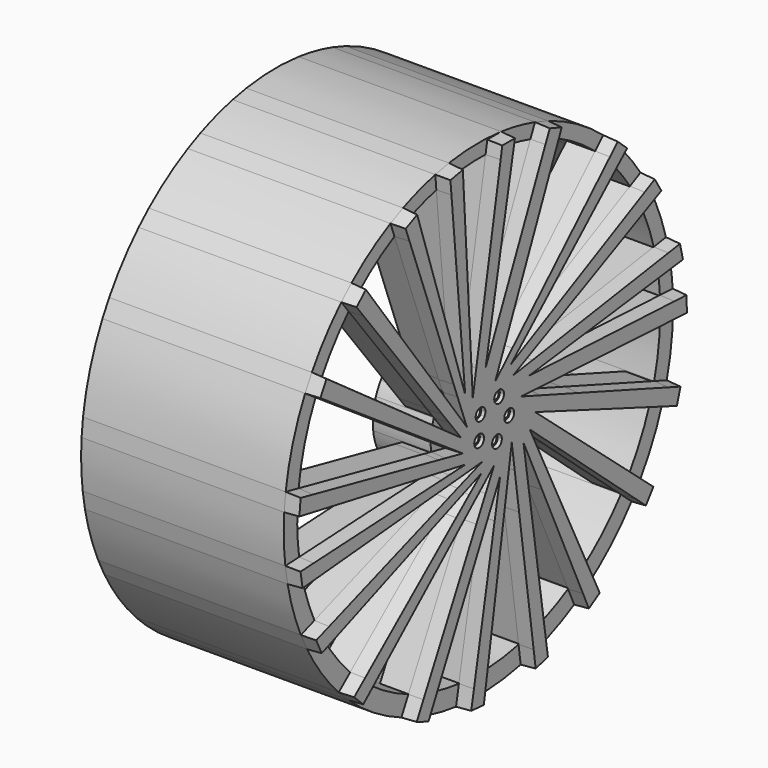
from build123d import *

# Parameters (mm, degrees)
F1_DEPTH               = 0.508
DRAFT_F1_DRAFTED_ANGLE = 3
F0_R                   = 0.1327768883
F2_DEPTH               = 0.381
F3_DEPTH               = 7.112
F4_DEPTH               = 2.032
F5_DEPTH               = 1.524


# Not quite as in the source:
# - an extrude with a draft is written as a straight extrude whose walls are then drafted


with BuildPart() as f1:
    # F0 (on Right) → F1 (new body)
    with BuildSketch(Plane.YZ):
        with BuildLine():
            ThreePointArc((2.0973634312, 0.1994440358), (2.0479166203, 0.4947209338), (1.9571150587, 0.7800076492))
            Line((1.9571150587, 0.7800076492), (1.874030917, 0.7837941521))
            Line((1.874030917, 0.7837941521), (1.9516786896, 0.7935121792))
            ThreePointArc((1.9516786896, 0.7935121792), (1.8474088258, 1.0128138607), (1.7185973208, 1.2186609598))
            Line((1.7185973208, 1.2186609598), (1.0488089186, 1.118784594))
            Line((1.0488089186, 1.118784594), (1.5952065231, 1.3762366928))
            ThreePointArc((1.5952065231, 1.3762366928), (1.4233301415, 1.5533327378), (1.2319239448, 1.7091151746))
            Line((1.2319239448, 1.7091151746), (0.9497648582, 1.5682294598))
            Line((0.9497648582, 1.5682294598), (1.1604227369, 1.7584454378))
            ThreePointArc((1.1604227369, 1.7584454378), (0.9931503964, 1.8580537065), (0.8173976146, 1.9417961854))
            Line((0.8173976146, 1.9417961854), (0.1672281942, 1.3095261529))
            Line((0.1672281942, 1.3095261529), (0.4908475213, 2.0488484563))
            ThreePointArc((0.4908475213, 2.0488484563), (0.1341704883, 2.1025483505), (-0.2264391893, 2.0946208678))
            Line((-0.2264391893, 2.0946208678), (-0.2628028451, 2.0138535183))
            Line((-0.2628028451, 2.0138535183), (-0.247458392, 2.0922417715))
            ThreePointArc((-0.247458392, 2.0922417715), (-0.5116791286, 2.0437455212), (-0.7675809957, 1.962022095))
            Line((-0.7675809957, 1.962022095), (-0.8833207471, 1.3116621244))
            Line((-0.8833207471, 1.3116621244), (-0.9184916182, 1.8960707881))
            ThreePointArc((-0.9184916182, 1.8960707881), (-1.108910163, 1.7913764363), (-1.2875318419, 1.6676249705))
            Line((-1.2875318419, 1.6676249705), (-1.278315313, 1.5696064409))
            Line((-1.278315313, 1.5696064409), (-1.3058418432, 1.653326455))
            ThreePointArc((-1.3058418432, 1.653326455), (-1.4535485576, 1.5250927437), (-1.588725858, 1.3837129161))
            Line((-1.588725858, 1.3837129161), (-1.2479530415, 0.4675828968))
            Line((-1.2479530415, 0.4675828968), (-1.7571567546, 1.1623731869))
            ThreePointArc((-1.7571567546, 1.1623731869), (-1.8749948406, 0.9607838643), (-1.9698009376, 0.7473925021))
            Line((-1.9698009376, 0.7473925021), (-1.5407761435, 0.1956446023))
            Line((-1.5407761435, 0.1956446023), (-2.0342080206, 0.5483694146))
            ThreePointArc((-2.0342080206, 0.5483694146), (-2.085479797, 0.2991409406), (-2.1063324905, 0.0455491574))
            Line((-2.1063324905, 0.0455491574), (-1.4629171928, -0.3922739706))
            Line((-1.4629171928, -0.3922739706), (-2.0909273042, -0.2583298172))
            ThreePointArc((-2.0909273042, -0.2583298172), (-2.0481428196, -0.4937836333), (-1.9789328462, -0.7228665687))
            Line((-1.9789328462, -0.7228665687), (-1.4450035524, -0.8222024771))
            Line((-1.4450035524, -0.8222024771), (-1.9290997886, -0.8469269695))
            ThreePointArc((-1.9290997886, -0.8469269695), (-1.8417203072, -1.0231214963), (-1.7382917618, -1.1904003683))
            Line((-1.7382917618, -1.1904003683), (-0.6942516193, -1.0973911267))
            Line((-0.6942516193, -1.0973911267), (-1.5700228728, -1.4048983824))
            ThreePointArc((-1.5700228728, -1.4048983824), (-1.4142027393, -1.5616471747), (-1.2428186419, -1.7012093079))
            Line((-1.2428186419, -1.7012093079), (-0.6553439889, -1.473498065))
            Line((-0.6553439889, -1.473498065), (-1.0673164667, -1.8164654816))
            ThreePointArc((-1.0673164667, -1.8164654816), (-0.8596663243, -1.9234565493), (-0.6414481891, -2.0068023088))
            Line((-0.6414481891, -2.0068023088), (-0.0466870831, -1.4831608295))
            Line((-0.0466870831, -1.4831608295), (-0.3546647591, -2.0767580973))
            ThreePointArc((-0.3546647591, -2.0767580973), (-0.0798113957, -2.1053126673), (0.1964149737, -2.0976492662))
            Line((0.1964149737, -2.0976492662), (0.241613948, -2.0070695918))
            Line((0.241613948, -2.0070695918), (0.2250988259, -2.094765334))
            ThreePointArc((0.2250988259, -2.094765334), (0.4544351286, -2.0572311489), (0.6782425081, -1.9946674876))
            Line((0.6782425081, -1.9946674876), (0.8121209103, -1.1625625193))
            Line((0.8121209103, -1.1625625193), (0.9161377334, -1.8972092503))
            ThreePointArc((0.9161377334, -1.8972092503), (1.175554891, -1.7483655179), (1.4112815226, -1.5642876175))
            Line((1.4112815226, -1.5642876175), (1.3831191463, -1.3788056094))
            Line((1.3831191463, -1.3788056094), (1.4509616475, -1.527554118))
            ThreePointArc((1.4509616475, -1.527554118), (1.6151213458, -1.3528097887), (1.7583642489, -1.1605457571))
            Line((1.7583642489, -1.1605457571), (1.6812520346, -1.0023429076))
            Line((1.6812520346, -1.0023429076), (1.795782543, -1.1017605657))
            ThreePointArc((1.795782543, -1.1017605657), (1.9279480867, -0.8495454439), (2.0248965585, -0.5818120085))
            Line((2.0248965585, -0.5818120085), (1.976531, -0.5406407308))
            Line((1.976531, -0.5406407308), (2.0307593005, -0.5610061939))
            ThreePointArc((2.0307593005, -0.5610061939), (2.0863309732, -0.2931456231), (2.1067267184, -0.0203425628))
            Line((2.1067267184, -0.0203425628), (1.4032723848, 0.234704974))
            Line((1.4032723848, 0.234704974), (2.0973634312, 0.1994440358))
        make_face()
        with BuildLine():
            ThreePointArc((-0.4288348497, -0.3488957607), (-0.7994075328, -0.396824389), (-0.4532226045, -0.2561927344))
            ThreePointArc((-0.4532226045, -0.2561927344), (-0.4350337778, -0.3009671323), (-0.4288348497, -0.3488957607))
        make_face(mode=Mode.SUBTRACT)
        with BuildLine():
            ThreePointArc((0.3531737773, -0.6895901054), (0.0480815647, -0.8374712276), (0.1210031397, -0.5063631963))
            ThreePointArc((0.1210031397, -0.5063631963), (0.2814943788, -0.5417089833), (0.3531737773, -0.6895901054))
        make_face(mode=Mode.SUBTRACT)
        with BuildLine():
            ThreePointArc((0.8904525658, -0.098953794), (0.6888882585, -0.2868780842), (0.515524755, -0.072661361))
            ThreePointArc((0.515524755, -0.072661361), (0.715245262, 0.0889704962), (0.8904525658, -0.098953794))
        make_face(mode=Mode.SUBTRACT)
        with BuildLine():
            ThreePointArc((-0.3656586917, 0.4424073736), (-0.3762498951, 0.3801314457), (-0.4068326133, 0.3248579246))
            ThreePointArc((-0.4068326133, 0.3248579246), (-0.7318390994, 0.5046833014), (-0.3656586917, 0.4424073736))
        make_face(mode=Mode.SUBTRACT)
        with BuildLine():
            ThreePointArc((0.1905582958, 0.4844924997), (0.430263846, 0.2931185242), (0.5206202516, 0))
            ThreePointArc((0.5206202516, 0), (0.5193448151, -0.0364199035), (0.515524755, -0.072661361))
            ThreePointArc((0.515524755, -0.072661361), (0.3851185021, -0.3503272552), (0.1210031397, -0.5063631963))
            ThreePointArc((0.1210031397, -0.5063631963), (-0.2079393137, -0.477290989), (-0.4532226045, -0.2561927344))
            ThreePointArc((-0.4532226045, -0.2561927344), (-0.5189688926, 0.0414334998), (-0.4068326133, 0.3248579246))
            ThreePointArc((-0.4068326133, 0.3248579246), (-0.1344040345, 0.5029721681), (0.1905582958, 0.4844924997))
        make_face(mode=Mode.SUBTRACT)
        with BuildLine():
            ThreePointArc((0.4478973964, 0.6598055194), (0.3655761695, 0.5041150672), (0.1905582958, 0.4844924997))
            ThreePointArc((0.1905582958, 0.4844924997), (0.1534470121, 0.8154959715), (0.4478973964, 0.6598055194))
        make_face(mode=Mode.SUBTRACT)
        with BuildLine():
            Line((1.5952065231, 1.3762366928), (6.9449263444, 3.8969223335))
            ThreePointArc((6.9449263444, 3.8969223335), (6.7939909706, 4.1544785827), (6.6335084956, 4.4061968454))
            Line((6.6335084956, 4.4061968454), (1.2319239448, 1.7091151746))
            ThreePointArc((1.2319239448, 1.7091151746), (1.4233301415, 1.5533327378), (1.5952065231, 1.3762366928))
        make_face()
        with BuildLine():
            Line((1.1604227369, 1.7584454378), (5.5440939511, 5.7167322715))
            ThreePointArc((5.5440939511, 5.7167322715), (5.3283953495, 5.9182943997), (5.1053741179, 6.11172322))
            Line((5.1053741179, 6.11172322), (0.8173976146, 1.9417961854))
            ThreePointArc((0.8173976146, 1.9417961854), (0.9931503964, 1.8580537065), (1.1604227369, 1.7584454378))
        make_face()
        with BuildLine():
            Line((0.4908475213, 2.0488484563), (2.8491231491, 7.4364307892))
            ThreePointArc((2.8491231491, 7.4364307892), (2.5602141598, 7.5407764228), (2.2674959584, 7.6339025197))
            Line((2.2674959584, 7.6339025197), (-0.2264391893, 2.0946208678))
            ThreePointArc((-0.2264391893, 2.0946208678), (0.1341704883, 2.1025483505), (0.4908475213, 2.0488484563))
        make_face()
        with BuildLine():
            Line((-0.247458392, 2.0922417715), (0.8920345152, 7.9134240393))
            ThreePointArc((0.8920345152, 7.9134240393), (0.5961637235, 7.9411960319), (0.2994627622, 7.9579097542))
            Line((0.2994627622, 7.9579097542), (-0.7675809957, 1.962022095))
            ThreePointArc((-0.7675809957, 1.962022095), (-0.5116791286, 2.0437455212), (-0.247458392, 2.0922417715))
        make_face()
        with BuildLine():
            Line((1.9516786896, 0.7935121792), (7.815688204, 1.5274238113))
            ThreePointArc((7.815688204, 1.5274238113), (7.7530721949, 1.8187570323), (7.6796005885, 2.1075436894))
            Line((7.6796005885, 2.1075436894), (1.7185973208, 1.2186609598))
            ThreePointArc((1.7185973208, 1.2186609598), (1.8474088258, 1.0128138607), (1.9516786896, 0.7935121792))
        make_face()
        with BuildLine():
            ThreePointArc((7.9635422773, 0), (7.9595022959, 0.253631237), (7.9473864506, 0.5070051349))
            Line((7.9473864506, 0.5070051349), (1.9571150587, 0.7800076492))
            ThreePointArc((1.9571150587, 0.7800076492), (2.0479166203, 0.4947209338), (2.0973634312, 0.1994440358))
            Line((2.0973634312, 0.1994440358), (7.9629326383, -0.098536286))
            ThreePointArc((7.9629326383, -0.098536286), (7.9633898661, -0.0492690859), (7.9635422773, 0))
        make_face()
        with BuildLine():
            Line((3.6408678629, -1.1656832036), (3.7447208571, -0.6142210141))
            Line((3.7447208571, -0.6142210141), (2.1067267184, -0.0203425628))
            ThreePointArc((2.1067267184, -0.0203425628), (2.0863309732, -0.2931456231), (2.0307593005, -0.5610061939))
            Line((2.0307593005, -0.5610061939), (3.6408678629, -1.1656832036))
        make_face()
        with BuildLine():
            Line((3.072494338, -2.2100041114), (3.4359816149, -1.7830009641))
            Line((3.4359816148, -1.7830009642), (2.0248965585, -0.5818120085))
            ThreePointArc((2.0248965585, -0.5818120085), (1.9279480867, -0.8495454439), (1.795782543, -1.1017605657))
            Line((1.795782543, -1.1017605657), (3.072494338, -2.2100041114))
        make_face()
        with BuildLine():
            Line((2.1177585519, -2.989543922), (2.5477149816, -2.7799718918))
            Line((2.5477149816, -2.7799718918), (1.7583642489, -1.1605457571))
            ThreePointArc((1.7583642489, -1.1605457571), (1.6151213458, -1.3528097887), (1.4509616475, -1.527554118))
            Line((1.4509616475, -1.527554118), (2.1177585519, -2.989543922))
        make_face()
        with BuildLine():
            Line((1.1092551824, -3.2611530648), (1.6571441187, -3.1835788183))
            Line((1.6571441187, -3.1835788183), (1.4112815226, -1.5642876175))
            ThreePointArc((1.4112815226, -1.5642876175), (1.175554891, -1.7483655179), (0.9161377334, -1.8972092503))
            Line((0.9161377334, -1.8972092503), (1.1092551824, -3.2611530648))
        make_face()
        with BuildLine():
            Line((0.0371511227, -3.092772688), (0.4879092453, -3.1776607938))
            Line((0.4879092453, -3.1776607938), (0.6782425081, -1.9946674876))
            ThreePointArc((0.6782425081, -1.9946674876), (0.4544351286, -2.0572311489), (0.2250988259, -2.094765334))
            Line((0.2250988259, -2.094765334), (0.0371511227, -3.092772688))
        make_face()
        with BuildLine():
            Line((-0.7621865916, -2.8622171261), (-0.3001485015, -3.092772688))
            Line((-0.3001485015, -3.092772688), (0.1964149737, -2.0976492662))
            ThreePointArc((0.1964149737, -2.0976492662), (-0.0798113957, -2.1053126673), (-0.3546647591, -2.0767580973))
            Line((-0.3546647591, -2.0767580973), (-0.7621865916, -2.8622171261))
        make_face()
        with BuildLine():
            Line((-1.6438714141, -2.2964479357), (-1.3590403138, -2.6385870674))
            Line((-1.3590403138, -2.6385870674), (-0.6414481891, -2.0068023088))
            ThreePointArc((-0.6414481891, -2.0068023088), (-0.8596663243, -1.9234565493), (-1.0673164667, -1.8164654816))
            Line((-1.0673164667, -1.8164654816), (-1.6438714141, -2.2964479357))
        make_face()
        with BuildLine():
            Line((-2.0013750129, -1.5563579243), (-1.865734508, -1.9426579311))
            Line((-1.865734508, -1.9426579311), (-1.2428186419, -1.7012093079))
            ThreePointArc((-1.2428186419, -1.7012093079), (-1.4142027393, -1.5616471747), (-1.5700228728, -1.4048983824))
            Line((-1.5700228728, -1.4048983824), (-2.0013750129, -1.5563579243))
        make_face()
        with BuildLine():
            Line((-2.2486883972, -0.8632494805), (-2.2297435834, -1.2341817895))
            Line((-2.2297435834, -1.2341817895), (-1.7382917618, -1.1904003683))
            ThreePointArc((-1.7382917618, -1.1904003683), (-1.8417203072, -1.0231214963), (-1.9290997886, -0.8469269695))
            Line((-1.9290997886, -0.8469269695), (-2.2486883972, -0.8632494805))
        make_face()
        with BuildLine():
            Line((-2.396198928, -0.1932204368), (-7.9028562959, 0.9812583594))
            ThreePointArc((-7.9028562959, 0.9812583594), (-7.9339836035, 0.685499658), (-7.9540462566, 0.3887849655))
            Line((-7.9540462566, 0.3887849655), (-1.9789328462, -0.7228665687))
            ThreePointArc((-1.9789328462, -0.7228665687), (-2.0481428196, -0.4937836333), (-2.0909273042, -0.2583298172))
            Line((-2.0909273042, -0.2583298172), (-2.396198928, -0.1932204368))
        make_face()
        with BuildLine():
            Line((-2.0342080206, 0.5483694146), (-2.3296303896, 0.7595491225))
            Line((-2.3296303896, 0.7595491225), (-2.5999285065, 0.38142515))
            Line((-2.5999285065, 0.38142515), (-2.1063324905, 0.0455491574))
            ThreePointArc((-2.1063324905, 0.0455491574), (-2.085479797, 0.2991409406), (-2.0342080206, 0.5483694146))
        make_face()
        with BuildLine():
            Line((-1.7571567546, 1.1623731869), (-1.9127883143, 1.3747268947))
            Line((-1.9127883143, 1.3747268947), (-2.259829666, 1.1203843291))
            Line((-2.259829666, 1.1203843291), (-1.9698009376, 0.7473925021))
            ThreePointArc((-1.9698009376, 0.7473925021), (-1.8749948406, 0.9607838643), (-1.7571567546, 1.1623731869))
        make_face()
        with BuildLine():
            Line((-1.3058418432, 1.653326455), (-1.4061380248, 1.9583702689))
            Line((-1.4061380248, 1.9583702689), (-1.7592902425, 1.8422563949))
            Line((-1.7592902425, 1.8422563949), (-1.588725858, 1.3837129161))
            ThreePointArc((-1.588725858, 1.3837129161), (-1.4535485576, 1.5250927437), (-1.3058418432, 1.653326455))
        make_face()
        with BuildLine():
            Line((-0.9184916182, 1.8960707881), (-1.2774377998, 7.8604171817))
            ThreePointArc((-1.2774377998, 7.8604171817), (-1.5692282722, 7.8074021436), (-1.8588424354, 7.7435592851))
            Line((-1.8588424354, 7.7435592851), (-1.2875318419, 1.6676249705))
            ThreePointArc((-1.2875318419, 1.6676249705), (-1.108910163, 1.7913764363), (-0.9184916182, 1.8960707881))
        make_face()
        with BuildLine():
            Line((8.5251259164, -0.127096606), (8.5059250158, 0.4815501224))
            Line((8.5059250158, 0.4815501224), (7.9473864506, 0.5070051349))
            ThreePointArc((7.9473864506, 0.5070051349), (7.9595022959, 0.253631237), (7.9635422773, 0))
            ThreePointArc((7.9635422773, 0), (7.9633898661, -0.0492690859), (7.9629326383, -0.098536286))
            Line((7.9629326383, -0.098536286), (8.5251259164, -0.127096606))
        make_face()
        with BuildLine():
            Line((7.815688204, 1.5274238113), (8.3569027992, 1.5951596644))
            Line((8.3569027992, 1.5951596644), (8.2153967808, 2.1874396331))
            Line((8.2153967808, 2.1874396331), (7.6796005885, 2.1075436894))
            ThreePointArc((7.6796005885, 2.1075436894), (7.7530721949, 1.8187570323), (7.815688204, 1.5274238113))
        make_face()
        with BuildLine():
            Line((6.9449263444, 3.8969223335), (7.4151328752, 4.1184746558))
            Line((7.4151328752, 4.1184746558), (7.0962027329, 4.6372261175))
            Line((7.0962027329, 4.6372261175), (6.6335084956, 4.4061968454))
            ThreePointArc((6.6335084956, 4.4061968454), (6.7939909706, 4.1544785827), (6.9449263444, 3.8969223335))
        make_face()
        with BuildLine():
            Line((5.5440939511, 5.7167322715), (5.9160746025, 6.0526165207))
            Line((5.9160746025, 6.0526165207), (5.4631233301, 6.4596234733))
            Line((5.4631233301, 6.4596234733), (5.1053741179, 6.11172322))
            ThreePointArc((5.1053741179, 6.11172322), (5.3283953495, 5.9182943997), (5.5440939511, 5.7167322715))
        make_face()
        with BuildLine():
            Line((2.8491231491, 7.4364307892), (3.0438867625, 7.8813766598))
            Line((3.0438867625, 7.8813766598), (2.4679152371, 8.0790539641))
            Line((2.4679152371, 8.0790539641), (2.2674959584, 7.6339025197))
            ThreePointArc((2.2674959584, 7.6339025197), (2.5602141598, 7.5407764228), (2.8491231491, 7.4364307892))
        make_face()
        with BuildLine():
            Line((0.8920345152, 7.9134240393), (0.9851502187, 8.3891123729))
            Line((0.9851502187, 8.3891123729), (0.3762007014, 8.3891123729))
            Line((0.3762007014, 8.3891123729), (0.2994627622, 7.9579097542))
            ThreePointArc((0.2994627622, 7.9579097542), (0.5961637235, 7.9411960319), (0.8920345152, 7.9134240393))
        make_face()
        with BuildLine():
            Line((-1.2774377998, 7.8604171817), (-1.3068695686, 8.3494633764))
            Line((-1.3068695686, 8.3494633764), (-1.9051367918, 8.2359035056))
            Line((-1.9051367918, 8.2359035056), (-1.8588424354, 7.7435592851))
            ThreePointArc((-1.8588424354, 7.7435592851), (-1.5692282722, 7.8074021436), (-1.2774377998, 7.8604171817))
        make_face()
        with BuildLine():
            Line((-3.1649303381, 7.3076139442), (-3.3208344512, 7.7817853883))
            Line((-3.3208344512, 7.7817853883), (-3.8735269928, 7.5261480101))
            Line((-3.8735269928, 7.5261480101), (-3.69756254, 7.053087045))
            ThreePointArc((-3.69756254, 7.053087045), (-3.4336057012, 7.1852875719), (-3.1649303381, 7.3076139442))
        make_face()
        with BuildLine():
            Line((-5.2765964735, 5.9645230537), (-5.5829759971, 6.3825669772))
            Line((-5.5829759971, 6.3825669772), (-6.0302049834, 5.9692804561))
            Line((-6.0302049834, 5.9692804561), (-5.7072115395, 5.5538943135))
            ThreePointArc((-5.7072115395, 5.5538943135), (-5.4957404967, 5.7632319054), (-5.2765964735, 5.9645230537))
        make_face()
        with BuildLine():
            Line((-6.8792189369, 4.0117767161), (-7.3214658744, 4.3279124893))
            Line((-7.3214658744, 4.3279124893), (-7.6178544375, 3.7959601096))
            Line((-7.6178544375, 3.7959601096), (-7.1605941762, 3.4848094132))
            ThreePointArc((-7.1605941762, 3.4848094132), (-7.0248495854, 3.7509324047), (-6.8792189369, 4.0117767161))
        make_face()
        with BuildLine():
            Line((-7.9028562959, 0.9812583594), (-8.4702794775, 1.1022803244))
            Line((-8.4702794775, 1.1022803244), (-8.5338796719, 0.496661195))
            Line((-8.5338796719, 0.496661195), (-7.9540462566, 0.3887849655))
            ThreePointArc((-7.9540462566, 0.3887849655), (-7.9339836035, 0.685499658), (-7.9028562959, 0.9812583594))
        make_face()
        with BuildLine():
            Line((-8.4843528563, -1.1817267316), (-8.385152521, -1.7825418514))
            Line((-8.385152521, -1.7825418514), (-7.7737862656, -1.7280777466))
            ThreePointArc((-7.7737862656, -1.7280777466), (-7.8321849534, -1.440445923), (-7.8799449627, -1.150857501))
            Line((-7.8799449627, -1.150857501), (-8.4843528563, -1.1817267316))
        make_face()
        with BuildLine():
            Line((-7.8032374756, -3.5935506237), (-7.5338954901, -4.1396956681))
            Line((-7.5338954901, -4.1396956681), (-6.9382405165, -3.9088136484))
            ThreePointArc((-6.9382405165, -3.9088136484), (-7.078198795, -3.6492612157), (-7.2084517805, -3.3847050877))
            Line((-7.2084517805, -3.3847050877), (-7.8032374756, -3.5935506237))
        make_face()
        with BuildLine():
            Line((-6.141372929, -6.0406215372), (-5.7018709735, -6.4621159568))
            Line((-5.7018709735, -6.4621159568), (-5.2064015452, -6.0258931746))
            ThreePointArc((-5.2064015452, -6.0258931746), (-5.426648368, -5.828335362), (-5.6394046273, -5.6227325253))
            Line((-5.6394046273, -5.6227325253), (-6.141372929, -6.0406215372))
        make_face()
        with BuildLine():
            Line((-3.3938361179, -7.9344677799), (-2.8263587751, -8.1553500565))
            Line((-2.8263587751, -8.1553500565), (-2.5255216294, -7.5524662264))
            ThreePointArc((-2.5255216294, -7.5524662264), (-2.8077795441, -7.4521392656), (-3.0860645148, -7.3412676979))
            Line((-3.0860645148, -7.3412676979), (-3.3938361179, -7.9344677799))
        make_face()
        with BuildLine():
            Line((-0.9952875843, -8.5750499622), (-0.3882586898, -8.6233763101))
            Line((-0.3882586898, -8.6233763101), (-0.2812975892, -7.9585725648))
            ThreePointArc((-0.2812975892, -7.9585725648), (-0.5766098133, -7.9426397832), (-0.8711268039, -7.9157528823))
            Line((-0.8711268039, -7.9157528823), (-0.9952875843, -8.5750499622))
        make_face()
        with BuildLine():
            Line((1.8407592491, -8.4275968658), (2.4300697842, -8.2741934502))
            Line((2.4300697842, -8.2741934502), (2.329991339, -7.61506047))
            ThreePointArc((2.329991339, -7.61506047), (2.0402414674, -7.6977542411), (1.7475706563, -7.769427418))
            Line((1.7475706563, -7.769427418), (1.8407592491, -8.4275968658))
        make_face()
        with BuildLine():
            Line((4.1870109951, -7.5264965599), (4.7061414243, -7.2081836445))
            Line((4.7061414243, -7.2081836445), (4.4211700232, -6.6235384221))
            ThreePointArc((4.4211700232, -6.6235384221), (4.1718143339, -6.7833598434), (3.9166881015, -6.9337983759))
            Line((3.9166881015, -6.9337983759), (4.1870109951, -7.5264965599))
        make_face()
        with BuildLine():
            Line((6.7044682025, -5.3627215915), (7.0630015105, -4.8705088513))
            Line((7.0630015105, -4.8705088513), (6.5913509419, -4.4690153684))
            ThreePointArc((6.5913509419, -4.4690153684), (6.4175056503, -4.7152546941), (6.2344663005, -4.9547386964))
            Line((6.2344663005, -4.9547386964), (6.7044682025, -5.3627215915))
        make_face()
        with BuildLine():
            Line((8.0741232887, -2.8305943137), (8.2487278584, -2.2472138556))
            Line((8.2487278584, -2.2472138556), (7.6960083248, -2.0468173994))
            ThreePointArc((7.6960083248, -2.0468173994), (7.6131533006, -2.3362154061), (7.5194200609, -2.6222752619))
            Line((7.5194200609, -2.6222752619), (8.0741232887, -2.8305943137))
        make_face()
        with BuildLine():
            ThreePointArc((0.515524755, -0.072661361), (0.5193448151, -0.0364199035), (0.5206202516, 0))
            ThreePointArc((0.5206202516, 0), (0.430263846, 0.2931185242), (0.1905582958, 0.4844924997))
            ThreePointArc((0.1905582958, 0.4844924997), (-0.1344040345, 0.5029721681), (-0.4068326133, 0.3248579246))
            ThreePointArc((-0.4068326133, 0.3248579246), (-0.5189688926, 0.0414334998), (-0.4532226045, -0.2561927344))
            ThreePointArc((-0.4532226045, -0.2561927344), (-0.2079393137, -0.477290989), (0.1210031397, -0.5063631963))
            ThreePointArc((0.1210031397, -0.5063631963), (0.3851185021, -0.3503272552), (0.515524755, -0.072661361))
        make_face()
        with BuildLine():
            ThreePointArc((7.5194200609, -2.6222752619), (7.6131533006, -2.3362154061), (7.6960083248, -2.0468173994))
            Line((7.6960083248, -2.0468173994), (3.7447208571, -0.6142210141))
            Line((3.7447208571, -0.6142210141), (3.6408678629, -1.1656832036))
            Line((3.6408678629, -1.1656832036), (7.5194200609, -2.6222752619))
        make_face()
        with BuildLine():
            ThreePointArc((6.2344663005, -4.9547386964), (6.4175056503, -4.7152546941), (6.5913509419, -4.4690153684))
            Line((6.5913509419, -4.4690153684), (3.4359816148, -1.7830009642))
            Line((3.4359816149, -1.7830009641), (3.072494338, -2.2100041114))
            Line((3.072494338, -2.2100041114), (6.2344663005, -4.9547386964))
        make_face()
        with BuildLine():
            ThreePointArc((3.9166881015, -6.9337983759), (4.1718143339, -6.7833598434), (4.4211700232, -6.6235384221))
            Line((4.4211700232, -6.6235384221), (2.5477149816, -2.7799718918))
            Line((2.5477149816, -2.7799718918), (2.1177585519, -2.989543922))
            Line((2.1177585519, -2.989543922), (3.9166881015, -6.9337983759))
        make_face()
        with BuildLine():
            ThreePointArc((1.7475706563, -7.769427418), (2.0402414674, -7.6977542411), (2.329991339, -7.61506047))
            Line((2.329991339, -7.61506047), (1.6571441187, -3.1835788183))
            Line((1.6571441187, -3.1835788183), (1.1092551824, -3.2611530648))
            Line((1.1092551824, -3.2611530648), (1.7475706563, -7.769427418))
        make_face()
        with BuildLine():
            ThreePointArc((-0.8711268039, -7.9157528823), (-0.5766098133, -7.9426397832), (-0.2812975892, -7.9585725648))
            Line((-0.2812975892, -7.9585725648), (0.4879092453, -3.1776607938))
            Line((0.4879092453, -3.1776607938), (0.0371511227, -3.092772688))
            Line((0.0371511227, -3.092772688), (-0.8711268039, -7.9157528823))
        make_face()
        with BuildLine():
            ThreePointArc((-3.0860645148, -7.3412676979), (-2.8077795441, -7.4521392656), (-2.5255216294, -7.5524662264))
            Line((-2.5255216294, -7.5524662264), (-0.3001485015, -3.092772688))
            Line((-0.3001485015, -3.092772688), (-0.7621865916, -2.8622171261))
            Line((-0.7621865916, -2.8622171261), (-3.0860645148, -7.3412676979))
        make_face()
        with BuildLine():
            ThreePointArc((-5.6394046273, -5.6227325253), (-5.426648368, -5.828335362), (-5.2064015452, -6.0258931746))
            Line((-5.2064015452, -6.0258931746), (-1.3590403138, -2.6385870674))
            Line((-1.3590403138, -2.6385870674), (-1.6438714141, -2.2964479357))
            Line((-1.6438714141, -2.2964479357), (-5.6394046273, -5.6227325253))
        make_face()
        with BuildLine():
            ThreePointArc((-7.2084517805, -3.3847050877), (-7.078198795, -3.6492612157), (-6.9382405165, -3.9088136484))
            Line((-6.9382405165, -3.9088136484), (-1.865734508, -1.9426579311))
            Line((-1.865734508, -1.9426579311), (-2.0013750129, -1.5563579243))
            Line((-2.0013750129, -1.5563579243), (-7.2084517805, -3.3847050877))
        make_face()
        with BuildLine():
            ThreePointArc((-7.8799449627, -1.150857501), (-7.8321849534, -1.440445923), (-7.7737862656, -1.7280777466))
            Line((-7.7737862656, -1.7280777466), (-2.2297435834, -1.2341817895))
            Line((-2.2297435834, -1.2341817895), (-2.2486883972, -0.8632494805))
            Line((-2.2486883972, -0.8632494805), (-7.8799449627, -1.150857501))
        make_face()
        with BuildLine():
            Line((-2.3296303896, 0.7595491225), (-6.8792189369, 4.0117767161))
            ThreePointArc((-6.8792189369, 4.0117767161), (-7.0248495854, 3.7509324047), (-7.1605941762, 3.4848094132))
            Line((-7.1605941762, 3.4848094132), (-2.5999285065, 0.38142515))
            Line((-2.5999285065, 0.38142515), (-2.3296303896, 0.7595491225))
        make_face()
        with BuildLine():
            Line((-1.9127883143, 1.3747268947), (-5.2765964735, 5.9645230537))
            ThreePointArc((-5.2765964735, 5.9645230537), (-5.4957404967, 5.7632319054), (-5.7072115395, 5.5538943135))
            Line((-5.7072115395, 5.5538943135), (-2.259829666, 1.1203843291))
            Line((-2.259829666, 1.1203843291), (-1.9127883143, 1.3747268947))
        make_face()
        with BuildLine():
            Line((-1.4061380248, 1.9583702689), (-3.1649303381, 7.3076139442))
            ThreePointArc((-3.1649303381, 7.3076139442), (-3.4336057012, 7.1852875719), (-3.69756254, 7.053087045))
            Line((-3.69756254, 7.053087045), (-1.7592902425, 1.8422563949))
            Line((-1.7592902425, 1.8422563949), (-1.4061380248, 1.9583702689))
        make_face()
    extrude(amount=F1_DEPTH)

    # draft_F1_drafted
    draft_f1_drafted_walls = [f1.faces().sort_by_distance(p)[0] for p in [
        (0.3386666667, 4.1928601186, -3.1825322496),
        (0.3386666667, 6.8837348565, -5.1166152214),
        (0.3386666667, 4.5197662553, -2.705574791),
        (0.3386666667, 5.0253271443, -1.6856175222),
        (0.3386666667, 8.1614255735, -2.5389040847),
        (0.3386666667, 4.8260001216, -1.0062544408),
        (0.3386666667, 4.9641991506, 0.053804184),
        (0.3386666667, 8.5155254661, 0.1772267582),
        (0.3386666667, 5.1899779664, 0.6326721373),
        (0.3386666667, 5.1154668581, 1.1894769082),
        (0.3386666667, 8.28614979, 1.8912996488),
        (0.3386666667, 4.6321028497, 1.6531121136),
        (0.3386666667, 4.2319708969, 2.6186296249),
        (0.3386666667, 7.255667804, 4.3778503866),
        (0.3386666667, 4.0229837956, 3.1027277886),
        (0.3386666667, 3.4329197304, 3.8104229903),
        (0.3386666667, 5.6895989663, 6.256119997),
        (0.3386666667, 2.8151757621, 3.8845748131),
        (0.3386666667, 1.6055574783, 4.5954514064),
        (0.3386666667, 2.7559009998, 7.980215312),
        (0.3386666667, 1.102556196, 5.0464537412),
        (0.3386666667, 0.3611736868, 5.2014829456),
        (0.3386666667, 0.68067546, 8.3891123729),
        (0.3386666667, -0.2535600228, 4.8503872487),
        (0.3386666667, -1.0950951578, 4.8305627504),
        (0.3386666667, -1.6060031802, 8.292683441),
        (0.3386666667, -1.5917260524, 4.9027549732),
        (0.3386666667, -2.2995748821, 4.6756959146),
        (0.3386666667, -3.597180722, 7.6539666992),
        (0.3386666667, -2.5607400171, 3.9968654535),
        (0.3386666667, -3.4154645193, 3.425074937),
        (0.3386666667, -5.8065904903, 6.1759237167),
        (0.3386666667, -3.7854905634, 3.0824625292),
        (0.3386666667, -4.4311210089, 2.2617785458),
        (0.3386666667, -7.469660156, 4.0619362994),
        (0.3386666667, -4.5403858152, 1.7018430695),
        (0.3386666667, -4.9665983352, 0.3550031769),
        (0.3386666667, -8.5020795747, 0.7994707597),
        (0.3386666667, -4.9894416121, -0.1627706411),
        (0.3386666667, -4.9646782043, -1.0019646044),
        (0.3386666667, -8.4347526886, -1.4821342915),
        (0.3386666667, -4.5397020701, -1.439966489),
        (0.3386666667, -4.2487445475, -2.3454708752),
        (0.3386666667, -7.6685664829, -3.8666231459),
        (0.3386666667, -4.0946197395, -2.8065968666),
        (0.3386666667, -3.398358459, -3.7570598011),
        (0.3386666667, -5.9216219513, -6.251368747),
        (0.3386666667, -2.8742790283, -3.9726383932),
        (0.3386666667, -1.7202616005, -4.7088143047),
        (0.3386666667, -3.1100974465, -8.0449089182),
        (0.3386666667, -1.2923724136, -5.0812098242),
        (0.3386666667, -0.3768368181, -5.291059777),
        (0.3386666667, -0.691773137, -8.5992131362),
        (0.3386666667, 0.2119311102, -4.8929694147),
        (0.3386666667, 1.3264400797, -4.7950796926),
        (0.3386666667, 2.1354145167, -8.350895158),
        (0.3386666667, 1.9065944653, -4.8264995298),
        (0.3386666667, 2.7850650707, -4.4526510847),
        (0.3386666667, 4.4465762097, -7.3673401022),
        (0.3386666667, 3.1936967295, -4.105263276),
        (0.3386666667, -0.7812187061, -0.4415987869),
        (0.3386666667, 0.2085728038, -0.8728170146),
        (0.3386666667, 0.8886087655, -0.125246227),
        (0.3386666667, -0.7012563813, 0.5599568225),
        (0.3386666667, 0.3284648859, 0.835118539),
    ]]
    draft(draft_f1_drafted_walls, neutral_plane=Plane.YZ, angle=DRAFT_F1_DRAFTED_ANGLE)


with BuildPart() as f2:
    # F0 (on Right) → F2 (new body)
    with BuildSketch(Plane.YZ):
        with BuildLine():
            ThreePointArc((0.4478973964, 0.6598055194), (0.1534470121, 0.8154959715), (0.1905582958, 0.4844924997))
            ThreePointArc((0.1905582958, 0.4844924997), (0.3655761695, 0.5041150672), (0.4478973964, 0.6598055194))
        make_face()
        with Locations((0.2595115908, 0.6598055194)):
            Circle(F0_R, mode=Mode.SUBTRACT)
    extrude(amount=F2_DEPTH)


with BuildPart() as f2b:
    # F0 (on Right) → F2, piece 2 (new body)
    with BuildSketch(Plane.YZ):
        with BuildLine():
            ThreePointArc((-0.3656586917, 0.4424073736), (-0.7318390994, 0.5046833014), (-0.4068326133, 0.3248579246))
            ThreePointArc((-0.4068326133, 0.3248579246), (-0.3762498951, 0.3801314457), (-0.3656586917, 0.4424073736))
        make_face()
        with Locations((-0.5540444973, 0.4424073736)):
            Circle(F0_R, mode=Mode.SUBTRACT)
    extrude(amount=F2_DEPTH)


with BuildPart() as f2c:
    # F0 (on Right) → F2, piece 3 (new body)
    with BuildSketch(Plane.YZ):
        with BuildLine():
            ThreePointArc((0.8904525658, -0.098953794), (0.715245262, 0.0889704962), (0.515524755, -0.072661361))
            ThreePointArc((0.515524755, -0.072661361), (0.6888882585, -0.2868780842), (0.8904525658, -0.098953794))
        make_face()
        with Locations((0.7020667602, -0.098953794)):
            Circle(F0_R, mode=Mode.SUBTRACT)
    extrude(amount=F2_DEPTH)


with BuildPart() as f2d:
    # F0 (on Right) → F2, piece 4 (new body)
    with BuildSketch(Plane.YZ):
        with BuildLine():
            ThreePointArc((0.3531737773, -0.6895901054), (0.2814943788, -0.5417089833), (0.1210031397, -0.5063631963))
            ThreePointArc((0.1210031397, -0.5063631963), (0.0480815647, -0.8374712276), (0.3531737773, -0.6895901054))
        make_face()
        with Locations((0.1647879717, -0.6895901054)):
            Circle(F0_R, mode=Mode.SUBTRACT)
    extrude(amount=F2_DEPTH)


with BuildPart() as f2e:
    # F0 (on Right) → F2, piece 5 (new body)
    with BuildSketch(Plane.YZ):
        with BuildLine():
            ThreePointArc((-0.4288348497, -0.3488957607), (-0.4350337778, -0.3009671323), (-0.4532226045, -0.2561927344))
            ThreePointArc((-0.4532226045, -0.2561927344), (-0.7994075328, -0.396824389), (-0.4288348497, -0.3488957607))
        make_face()
        with Locations((-0.6172206553, -0.3488957607)):
            Circle(F0_R, mode=Mode.SUBTRACT)
    extrude(amount=F2_DEPTH)


with BuildPart() as f3:
    # F0 (on Right) → F3 (new body)
    with BuildSketch(Plane.YZ):
        with BuildLine():
            Line((-3.69756254, 7.053087045), (-3.8735269928, 7.5261480101))
            ThreePointArc((-3.8735269928, 7.5261480101), (-4.7628046486, 7.0060082751), (-5.5829759971, 6.3825669772))
            Line((-5.5829759971, 6.3825669772), (-5.2765964735, 5.9645230537))
            ThreePointArc((-5.2765964735, 5.9645230537), (-4.5199696228, 6.556514334), (-3.69756254, 7.053087045))
        make_face()
        with BuildLine():
            Line((-5.2765964735, 5.9645230537), (-5.5829759971, 6.3825669772))
            Line((-5.5829759971, 6.3825669772), (-6.0302049834, 5.9692804561))
            Line((-6.0302049834, 5.9692804561), (-5.7072115395, 5.5538943135))
            ThreePointArc((-5.7072115395, 5.5538943135), (-5.4957404967, 5.7632319054), (-5.2765964735, 5.9645230537))
        make_face()
        with BuildLine():
            Line((-5.7072115395, 5.5538943135), (-6.0302049834, 5.9692804561))
            ThreePointArc((-6.0302049834, 5.9692804561), (-6.7261995721, 5.1882178432), (-7.3214658744, 4.3279124893))
            Line((-7.3214658744, 4.3279124893), (-6.8792189369, 4.0117767161))
            ThreePointArc((-6.8792189369, 4.0117767161), (-6.3402752074, 4.8186010311), (-5.7072115395, 5.5538943135))
        make_face()
        with BuildLine():
            Line((-6.8792189369, 4.0117767161), (-7.3214658744, 4.3279124893))
            Line((-7.3214658744, 4.3279124893), (-7.6178544375, 3.7959601096))
            Line((-7.6178544375, 3.7959601096), (-7.1605941762, 3.4848094132))
            ThreePointArc((-7.1605941762, 3.4848094132), (-7.0248495854, 3.7509324047), (-6.8792189369, 4.0117767161))
        make_face()
        with BuildLine():
            Line((-7.1605941762, 3.4848094132), (-7.6178544375, 3.7959601096))
            ThreePointArc((-7.6178544375, 3.7959601096), (-8.156239467, 2.4846176271), (-8.4702794775, 1.1022803244))
            Line((-8.4702794775, 1.1022803244), (-7.9028562959, 0.9812583594))
            ThreePointArc((-7.9028562959, 0.9812583594), (-7.6350394237, 2.2636648606), (-7.1605941762, 3.4848094132))
        make_face()
        with BuildLine():
            Line((-7.9028562959, 0.9812583594), (-8.4702794775, 1.1022803244))
            Line((-8.4702794775, 1.1022803244), (-8.5338796719, 0.496661195))
            Line((-8.5338796719, 0.496661195), (-7.9540462566, 0.3887849655))
            ThreePointArc((-7.9540462566, 0.3887849655), (-7.9339836035, 0.685499658), (-7.9028562959, 0.9812583594))
        make_face()
        with BuildLine():
            ThreePointArc((-8.5338796719, 0.496661195), (-8.5504680977, -0.3437530015), (-8.4843528563, -1.1817267316))
            Line((-8.4843528563, -1.1817267316), (-7.8799449627, -1.150857501))
            ThreePointArc((-7.8799449627, -1.150857501), (-7.9543349322, -0.3828333682), (-7.9540462566, 0.3887849655))
            Line((-7.9540462566, 0.3887849655), (-8.5338796719, 0.496661195))
        make_face()
        with BuildLine():
            Line((-8.4843528563, -1.1817267316), (-8.385152521, -1.7825418514))
            Line((-8.385152521, -1.7825418514), (-7.7737862656, -1.7280777466))
            ThreePointArc((-7.7737862656, -1.7280777466), (-7.8321849534, -1.440445923), (-7.8799449627, -1.150857501))
            Line((-7.8799449627, -1.150857501), (-8.4843528563, -1.1817267316))
        make_face()
        with BuildLine():
            ThreePointArc((-8.385152521, -1.7825418514), (-8.1447772834, -2.7042993851), (-7.8032374756, -3.5935506237))
            Line((-7.8032374756, -3.5935506237), (-7.2084517805, -3.3847050877))
            ThreePointArc((-7.2084517805, -3.3847050877), (-7.5367743601, -2.5719715876), (-7.7737862656, -1.7280777466))
            Line((-7.7737862656, -1.7280777466), (-8.385152521, -1.7825418514))
        make_face()
        with BuildLine():
            Line((-7.8032374756, -3.5935506237), (-7.5338954901, -4.1396956681))
            Line((-7.5338954901, -4.1396956681), (-6.9382405165, -3.9088136484))
            ThreePointArc((-6.9382405165, -3.9088136484), (-7.078198795, -3.6492612157), (-7.2084517805, -3.3847050877))
            Line((-7.2084517805, -3.3847050877), (-7.8032374756, -3.5935506237))
        make_face()
        with BuildLine():
            ThreePointArc((-7.5338954901, -4.1396956681), (-6.9035158404, -5.1384201676), (-6.141372929, -6.0406215372))
            Line((-6.141372929, -6.0406215372), (-5.6394046273, -5.6227325253))
            ThreePointArc((-5.6394046273, -5.6227325253), (-6.3469416903, -4.8098167098), (-6.9382405165, -3.9088136484))
            Line((-6.9382405165, -3.9088136484), (-7.5338954901, -4.1396956681))
        make_face()
        with BuildLine():
            Line((-6.141372929, -6.0406215372), (-5.7018709735, -6.4621159568))
            Line((-5.7018709735, -6.4621159568), (-5.2064015452, -6.0258931746))
            ThreePointArc((-5.2064015452, -6.0258931746), (-5.426648368, -5.828335362), (-5.6394046273, -5.6227325253))
            Line((-5.6394046273, -5.6227325253), (-6.141372929, -6.0406215372))
        make_face()
        with BuildLine():
            ThreePointArc((-5.7018709735, -6.4621159568), (-4.6072386663, -7.291383021), (-3.3938361179, -7.9344677799))
            Line((-3.3938361179, -7.9344677799), (-3.0860645148, -7.3412676979))
            ThreePointArc((-3.0860645148, -7.3412676979), (-4.1980710896, -6.7671415479), (-5.2064015452, -6.0258931746))
            Line((-5.2064015452, -6.0258931746), (-5.7018709735, -6.4621159568))
        make_face()
        with BuildLine():
            Line((-3.3938361179, -7.9344677799), (-2.8263587751, -8.1553500565))
            Line((-2.8263587751, -8.1553500565), (-2.5255216294, -7.5524662264))
            ThreePointArc((-2.5255216294, -7.5524662264), (-2.8077795441, -7.4521392656), (-3.0860645148, -7.3412676979))
            Line((-3.0860645148, -7.3412676979), (-3.3938361179, -7.9344677799))
        make_face()
        with BuildLine():
            ThreePointArc((-2.8263587751, -8.1553500565), (-1.9223989575, -8.4157029351), (-0.9952875843, -8.5750499622))
            Line((-0.9952875843, -8.5750499622), (-0.8711268039, -7.9157528823))
            ThreePointArc((-0.8711268039, -7.9157528823), (-1.7080103757, -7.7782199865), (-2.5255216294, -7.5524662264))
            Line((-2.5255216294, -7.5524662264), (-2.8263587751, -8.1553500565))
        make_face()
        with BuildLine():
            Line((-3.1649303381, 7.3076139442), (-3.3208344512, 7.7817853883))
            Line((-3.3208344512, 7.7817853883), (-3.8735269928, 7.5261480101))
            Line((-3.8735269928, 7.5261480101), (-3.69756254, 7.053087045))
            ThreePointArc((-3.69756254, 7.053087045), (-3.4336057012, 7.1852875719), (-3.1649303381, 7.3076139442))
        make_face()
        with BuildLine():
            Line((-1.8588424354, 7.7435592851), (-1.9051367918, 8.2359035056))
            ThreePointArc((-1.9051367918, 8.2359035056), (-2.6228870866, 8.0397119249), (-3.3208344512, 7.7817853883))
            Line((-3.3208344512, 7.7817853883), (-3.1649303381, 7.3076139442))
            ThreePointArc((-3.1649303381, 7.3076139442), (-2.5213261005, 7.5538679031), (-1.8588424354, 7.7435592851))
        make_face()
        with BuildLine():
            Line((-1.2774377998, 7.8604171817), (-1.3068695686, 8.3494633764))
            Line((-1.3068695686, 8.3494633764), (-1.9051367918, 8.2359035056))
            Line((-1.9051367918, 8.2359035056), (-1.8588424354, 7.7435592851))
            ThreePointArc((-1.8588424354, 7.7435592851), (-1.5692282722, 7.8074021436), (-1.2774377998, 7.8604171817))
        make_face()
        with BuildLine():
            Line((0.3762007014, 8.3891123729), (0.9851502187, 8.3891123729))
            ThreePointArc((0.9851502187, 8.3891123729), (-0.1621961247, 8.4465450443), (-1.3068695686, 8.3494633764))
            Line((-1.3068695686, 8.3494633764), (-1.2774377998, 7.8604171817))
            ThreePointArc((-1.2774377998, 7.8604171817), (-0.4914112269, 7.948365908), (0.2994627622, 7.9579097542))
            Line((0.2994627622, 7.9579097542), (0.3762007014, 8.3891123729))
        make_face()
        with BuildLine():
            Line((0.8920345152, 7.9134240393), (0.9851502187, 8.3891123729))
            Line((0.9851502187, 8.3891123729), (0.3762007014, 8.3891123729))
            Line((0.3762007014, 8.3891123729), (0.2994627622, 7.9579097542))
            ThreePointArc((0.2994627622, 7.9579097542), (0.5961637235, 7.9411960319), (0.8920345152, 7.9134240393))
        make_face()
        with BuildLine():
            Line((2.2674959584, 7.6339025197), (2.4679152371, 8.0790539641))
            ThreePointArc((2.4679152371, 8.0790539641), (1.7334213703, 8.2670261161), (0.9851502187, 8.3891123729))
            Line((0.9851502187, 8.3891123729), (0.8920345152, 7.9134240393))
            ThreePointArc((0.8920345152, 7.9134240393), (1.5859354569, 7.8040255208), (2.2674959584, 7.6339025197))
        make_face()
        with BuildLine():
            Line((2.8491231491, 7.4364307892), (3.0438867625, 7.8813766598))
            Line((3.0438867625, 7.8813766598), (2.4679152371, 8.0790539641))
            Line((2.4679152371, 8.0790539641), (2.2674959584, 7.6339025197))
            ThreePointArc((2.2674959584, 7.6339025197), (2.5602141598, 7.5407764228), (2.8491231491, 7.4364307892))
        make_face()
        with BuildLine():
            Line((5.1053741179, 6.11172322), (5.4631233301, 6.4596234733))
            ThreePointArc((5.4631233301, 6.4596234733), (4.3123017615, 7.2705477857), (3.0438867625, 7.8813766598))
            Line((3.0438867625, 7.8813766598), (2.8491231491, 7.4364307892))
            ThreePointArc((2.8491231491, 7.4364307892), (4.0320242098, 6.8673711399), (5.1053741179, 6.11172322))
        make_face()
        with BuildLine():
            Line((5.5440939511, 5.7167322715), (5.9160746025, 6.0526165207))
            Line((5.9160746025, 6.0526165207), (5.4631233301, 6.4596234733))
            Line((5.4631233301, 6.4596234733), (5.1053741179, 6.11172322))
            ThreePointArc((5.1053741179, 6.11172322), (5.3283953495, 5.9182943997), (5.5440939511, 5.7167322715))
        make_face()
        with BuildLine():
            Line((6.6335084956, 4.4061968454), (7.0962027329, 4.6372261175))
            ThreePointArc((7.0962027329, 4.6372261175), (6.5444299207, 5.376847906), (5.9160746025, 6.0526165207))
            Line((5.9160746025, 6.0526165207), (5.5440939511, 5.7167322715))
            ThreePointArc((5.5440939511, 5.7167322715), (6.1239591861, 5.0906904727), (6.6335084956, 4.4061968454))
        make_face()
        with BuildLine():
            Line((6.9449263444, 3.8969223335), (7.4151328752, 4.1184746558))
            Line((7.4151328752, 4.1184746558), (7.0962027329, 4.6372261175))
            Line((7.0962027329, 4.6372261175), (6.6335084956, 4.4061968454))
            ThreePointArc((6.6335084956, 4.4061968454), (6.7939909706, 4.1544785827), (6.9449263444, 3.8969223335))
        make_face()
        with BuildLine():
            Line((7.6796005885, 2.1075436894), (8.2153967808, 2.1874396331))
            ThreePointArc((8.2153967808, 2.1874396331), (7.8745710614, 3.177534968), (7.4151328752, 4.1184746558))
            Line((7.4151328752, 4.1184746558), (6.9449263444, 3.8969223335))
            ThreePointArc((6.9449263444, 3.8969223335), (7.3667948245, 3.024622227), (7.6796005885, 2.1075436894))
        make_face()
        with BuildLine():
            Line((7.815688204, 1.5274238113), (8.3569027992, 1.5951596644))
            Line((8.3569027992, 1.5951596644), (8.2153967808, 2.1874396331))
            Line((8.2153967808, 2.1874396331), (7.6796005885, 2.1075436894))
            ThreePointArc((7.6796005885, 2.1075436894), (7.7530721949, 1.8187570323), (7.815688204, 1.5274238113))
        make_face()
        with BuildLine():
            Line((7.9473864506, 0.5070051349), (8.5059250158, 0.4815501224))
            ThreePointArc((8.5059250158, 0.4815501224), (8.4497479619, 1.0408083399), (8.3569027992, 1.5951596644))
            Line((8.3569027992, 1.5951596644), (7.815688204, 1.5274238113))
            ThreePointArc((7.815688204, 1.5274238113), (7.8980341991, 1.0193436081), (7.9473864506, 0.5070051349))
        make_face()
        with BuildLine():
            Line((8.5251259164, -0.127096606), (8.5059250158, 0.4815501224))
            Line((8.5059250158, 0.4815501224), (7.9473864506, 0.5070051349))
            ThreePointArc((7.9473864506, 0.5070051349), (7.9595022959, 0.253631237), (7.9635422773, 0))
            ThreePointArc((7.9635422773, 0), (7.9633898661, -0.0492690859), (7.9629326383, -0.098536286))
            Line((7.9629326383, -0.098536286), (8.5251259164, -0.127096606))
        make_face()
        with BuildLine():
            ThreePointArc((8.2487278584, -2.2472138556), (8.4535398574, -1.1958395126), (8.5251259164, -0.127096606))
            Line((8.5251259164, -0.127096606), (7.9629326383, -0.098536286))
            ThreePointArc((7.9629326383, -0.098536286), (7.8898388986, -1.0809476195), (7.6960083248, -2.0468173994))
            Line((7.6960083248, -2.0468173994), (8.2487278584, -2.2472138556))
        make_face()
        with BuildLine():
            Line((8.0741232887, -2.8305943137), (8.2487278584, -2.2472138556))
            Line((8.2487278584, -2.2472138556), (7.6960083248, -2.0468173994))
            ThreePointArc((7.6960083248, -2.0468173994), (7.6131533006, -2.3362154061), (7.5194200609, -2.6222752619))
            Line((7.5194200609, -2.6222752619), (8.0741232887, -2.8305943137))
        make_face()
        with BuildLine():
            ThreePointArc((7.0630015105, -4.8705088513), (7.6368495022, -3.8843993616), (8.0741232887, -2.8305943137))
            Line((8.0741232887, -2.8305943137), (7.5194200609, -2.6222752619))
            ThreePointArc((7.5194200609, -2.6222752619), (7.1155517586, -3.5758815379), (6.5913509419, -4.4690153684))
            Line((6.5913509419, -4.4690153684), (7.0630015105, -4.8705088513))
        make_face()
        with BuildLine():
            Line((6.7044682025, -5.3627215915), (7.0630015105, -4.8705088513))
            Line((7.0630015105, -4.8705088513), (6.5913509419, -4.4690153684))
            ThreePointArc((6.5913509419, -4.4690153684), (6.4175056503, -4.7152546941), (6.2344663005, -4.9547386964))
            Line((6.2344663005, -4.9547386964), (6.7044682025, -5.3627215915))
        make_face()
        with BuildLine():
            ThreePointArc((4.7061414243, -7.2081836445), (5.7792553239, -6.3655286538), (6.7044682025, -5.3627215915))
            Line((6.7044682025, -5.3627215915), (6.2344663005, -4.9547386964))
            ThreePointArc((6.2344663005, -4.9547386964), (5.3927608418, -5.8597044384), (4.4211700232, -6.6235384221))
            Line((4.4211700232, -6.6235384221), (4.7061414243, -7.2081836445))
        make_face()
        with BuildLine():
            ThreePointArc((2.4300697842, -8.2741934502), (3.3295036489, -7.9496045574), (4.1870109951, -7.5264965599))
            Line((4.1870109951, -7.5264965599), (3.9166881015, -6.9337983759))
            ThreePointArc((3.9166881015, -6.9337983759), (3.1418594046, -7.317562783), (2.329991339, -7.61506047))
            Line((2.329991339, -7.61506047), (2.4300697842, -8.2741934502))
        make_face()
        with BuildLine():
            Line((4.1870109951, -7.5264965599), (4.7061414243, -7.2081836445))
            Line((4.7061414243, -7.2081836445), (4.4211700232, -6.6235384221))
            ThreePointArc((4.4211700232, -6.6235384221), (4.1718143339, -6.7833598434), (3.9166881015, -6.9337983759))
            Line((3.9166881015, -6.9337983759), (4.1870109951, -7.5264965599))
        make_face()
        with BuildLine():
            ThreePointArc((-0.3882586898, -8.6233763101), (0.7326903845, -8.5988094494), (1.8407592491, -8.4275968658))
            Line((1.8407592491, -8.4275968658), (1.7475706563, -7.769427418))
            ThreePointArc((1.7475706563, -7.769427418), (0.7392111663, -7.929159631), (-0.2812975892, -7.9585725648))
            Line((-0.2812975892, -7.9585725648), (-0.3882586898, -8.6233763101))
        make_face()
        with BuildLine():
            Line((1.8407592491, -8.4275968658), (2.4300697842, -8.2741934502))
            Line((2.4300697842, -8.2741934502), (2.329991339, -7.61506047))
            ThreePointArc((2.329991339, -7.61506047), (2.0402414674, -7.6977542411), (1.7475706563, -7.769427418))
            Line((1.7475706563, -7.769427418), (1.8407592491, -8.4275968658))
        make_face()
        with BuildLine():
            Line((-0.9952875843, -8.5750499622), (-0.3882586898, -8.6233763101))
            Line((-0.3882586898, -8.6233763101), (-0.2812975892, -7.9585725648))
            ThreePointArc((-0.2812975892, -7.9585725648), (-0.5766098133, -7.9426397832), (-0.8711268039, -7.9157528823))
            Line((-0.8711268039, -7.9157528823), (-0.9952875843, -8.5750499622))
        make_face()
    extrude(amount=-F3_DEPTH)


with BuildPart() as f4:
    # F0 (on Right) → F4 (new body)
    with BuildSketch(Plane.YZ):
        with BuildLine():
            ThreePointArc((2.0973634312, 0.1994440358), (2.0479166203, 0.4947209338), (1.9571150587, 0.7800076492))
            Line((1.9571150587, 0.7800076492), (1.874030917, 0.7837941521))
            Line((1.874030917, 0.7837941521), (1.9516786896, 0.7935121792))
            ThreePointArc((1.9516786896, 0.7935121792), (1.8474088258, 1.0128138607), (1.7185973208, 1.2186609598))
            Line((1.7185973208, 1.2186609598), (1.0488089186, 1.118784594))
            Line((1.0488089186, 1.118784594), (1.5952065231, 1.3762366928))
            ThreePointArc((1.5952065231, 1.3762366928), (1.4233301415, 1.5533327378), (1.2319239448, 1.7091151746))
            Line((1.2319239448, 1.7091151746), (0.9497648582, 1.5682294598))
            Line((0.9497648582, 1.5682294598), (1.1604227369, 1.7584454378))
            ThreePointArc((1.1604227369, 1.7584454378), (0.9931503964, 1.8580537065), (0.8173976146, 1.9417961854))
            Line((0.8173976146, 1.9417961854), (0.1672281942, 1.3095261529))
            Line((0.1672281942, 1.3095261529), (0.4908475213, 2.0488484563))
            ThreePointArc((0.4908475213, 2.0488484563), (0.1341704883, 2.1025483505), (-0.2264391893, 2.0946208678))
            Line((-0.2264391893, 2.0946208678), (-0.2628028451, 2.0138535183))
            Line((-0.2628028451, 2.0138535183), (-0.247458392, 2.0922417715))
            ThreePointArc((-0.247458392, 2.0922417715), (-0.5116791286, 2.0437455212), (-0.7675809957, 1.962022095))
            Line((-0.7675809957, 1.962022095), (-0.8833207471, 1.3116621244))
            Line((-0.8833207471, 1.3116621244), (-0.9184916182, 1.8960707881))
            ThreePointArc((-0.9184916182, 1.8960707881), (-1.108910163, 1.7913764363), (-1.2875318419, 1.6676249705))
            Line((-1.2875318419, 1.6676249705), (-1.278315313, 1.5696064409))
            Line((-1.278315313, 1.5696064409), (-1.3058418432, 1.653326455))
            ThreePointArc((-1.3058418432, 1.653326455), (-1.4535485576, 1.5250927437), (-1.588725858, 1.3837129161))
            Line((-1.588725858, 1.3837129161), (-1.2479530415, 0.4675828968))
            Line((-1.2479530415, 0.4675828968), (-1.7571567546, 1.1623731869))
            ThreePointArc((-1.7571567546, 1.1623731869), (-1.8749948406, 0.9607838643), (-1.9698009376, 0.7473925021))
            Line((-1.9698009376, 0.7473925021), (-1.5407761435, 0.1956446023))
            Line((-1.5407761435, 0.1956446023), (-2.0342080206, 0.5483694146))
            ThreePointArc((-2.0342080206, 0.5483694146), (-2.085479797, 0.2991409406), (-2.1063324905, 0.0455491574))
            Line((-2.1063324905, 0.0455491574), (-1.4629171928, -0.3922739706))
            Line((-1.4629171928, -0.3922739706), (-2.0909273042, -0.2583298172))
            ThreePointArc((-2.0909273042, -0.2583298172), (-2.0481428196, -0.4937836333), (-1.9789328462, -0.7228665687))
            Line((-1.9789328462, -0.7228665687), (-1.4450035524, -0.8222024771))
            Line((-1.4450035524, -0.8222024771), (-1.9290997886, -0.8469269695))
            ThreePointArc((-1.9290997886, -0.8469269695), (-1.8417203072, -1.0231214963), (-1.7382917618, -1.1904003683))
            Line((-1.7382917618, -1.1904003683), (-0.6942516193, -1.0973911267))
            Line((-0.6942516193, -1.0973911267), (-1.5700228728, -1.4048983824))
            ThreePointArc((-1.5700228728, -1.4048983824), (-1.4142027393, -1.5616471747), (-1.2428186419, -1.7012093079))
            Line((-1.2428186419, -1.7012093079), (-0.6553439889, -1.473498065))
            Line((-0.6553439889, -1.473498065), (-1.0673164667, -1.8164654816))
            ThreePointArc((-1.0673164667, -1.8164654816), (-0.8596663243, -1.9234565493), (-0.6414481891, -2.0068023088))
            Line((-0.6414481891, -2.0068023088), (-0.0466870831, -1.4831608295))
            Line((-0.0466870831, -1.4831608295), (-0.3546647591, -2.0767580973))
            ThreePointArc((-0.3546647591, -2.0767580973), (-0.0798113957, -2.1053126673), (0.1964149737, -2.0976492662))
            Line((0.1964149737, -2.0976492662), (0.241613948, -2.0070695918))
            Line((0.241613948, -2.0070695918), (0.2250988259, -2.094765334))
            ThreePointArc((0.2250988259, -2.094765334), (0.4544351286, -2.0572311489), (0.6782425081, -1.9946674876))
            Line((0.6782425081, -1.9946674876), (0.8121209103, -1.1625625193))
            Line((0.8121209103, -1.1625625193), (0.9161377334, -1.8972092503))
            ThreePointArc((0.9161377334, -1.8972092503), (1.175554891, -1.7483655179), (1.4112815226, -1.5642876175))
            Line((1.4112815226, -1.5642876175), (1.3831191463, -1.3788056094))
            Line((1.3831191463, -1.3788056094), (1.4509616475, -1.527554118))
            ThreePointArc((1.4509616475, -1.527554118), (1.6151213458, -1.3528097887), (1.7583642489, -1.1605457571))
            Line((1.7583642489, -1.1605457571), (1.6812520346, -1.0023429076))
            Line((1.6812520346, -1.0023429076), (1.795782543, -1.1017605657))
            ThreePointArc((1.795782543, -1.1017605657), (1.9279480867, -0.8495454439), (2.0248965585, -0.5818120085))
            Line((2.0248965585, -0.5818120085), (1.976531, -0.5406407308))
            Line((1.976531, -0.5406407308), (2.0307593005, -0.5610061939))
            ThreePointArc((2.0307593005, -0.5610061939), (2.0863309732, -0.2931456231), (2.1067267184, -0.0203425628))
            Line((2.1067267184, -0.0203425628), (1.4032723848, 0.234704974))
            Line((1.4032723848, 0.234704974), (2.0973634312, 0.1994440358))
        make_face()
        with BuildLine():
            ThreePointArc((-0.4288348497, -0.3488957607), (-0.7994075328, -0.396824389), (-0.4532226045, -0.2561927344))
            ThreePointArc((-0.4532226045, -0.2561927344), (-0.4350337778, -0.3009671323), (-0.4288348497, -0.3488957607))
        make_face(mode=Mode.SUBTRACT)
        with BuildLine():
            ThreePointArc((0.3531737773, -0.6895901054), (0.0480815647, -0.8374712276), (0.1210031397, -0.5063631963))
            ThreePointArc((0.1210031397, -0.5063631963), (0.2814943788, -0.5417089833), (0.3531737773, -0.6895901054))
        make_face(mode=Mode.SUBTRACT)
        with BuildLine():
            ThreePointArc((0.8904525658, -0.098953794), (0.6888882585, -0.2868780842), (0.515524755, -0.072661361))
            ThreePointArc((0.515524755, -0.072661361), (0.715245262, 0.0889704962), (0.8904525658, -0.098953794))
        make_face(mode=Mode.SUBTRACT)
        with BuildLine():
            ThreePointArc((-0.3656586917, 0.4424073736), (-0.3762498951, 0.3801314457), (-0.4068326133, 0.3248579246))
            ThreePointArc((-0.4068326133, 0.3248579246), (-0.7318390994, 0.5046833014), (-0.3656586917, 0.4424073736))
        make_face(mode=Mode.SUBTRACT)
        with BuildLine():
            ThreePointArc((0.1905582958, 0.4844924997), (0.430263846, 0.2931185242), (0.5206202516, 0))
            ThreePointArc((0.5206202516, 0), (0.5193448151, -0.0364199035), (0.515524755, -0.072661361))
            ThreePointArc((0.515524755, -0.072661361), (0.3851185021, -0.3503272552), (0.1210031397, -0.5063631963))
            ThreePointArc((0.1210031397, -0.5063631963), (-0.2079393137, -0.477290989), (-0.4532226045, -0.2561927344))
            ThreePointArc((-0.4532226045, -0.2561927344), (-0.5189688926, 0.0414334998), (-0.4068326133, 0.3248579246))
            ThreePointArc((-0.4068326133, 0.3248579246), (-0.1344040345, 0.5029721681), (0.1905582958, 0.4844924997))
        make_face(mode=Mode.SUBTRACT)
        with BuildLine():
            ThreePointArc((0.4478973964, 0.6598055194), (0.3655761695, 0.5041150672), (0.1905582958, 0.4844924997))
            ThreePointArc((0.1905582958, 0.4844924997), (0.1534470121, 0.8154959715), (0.4478973964, 0.6598055194))
        make_face(mode=Mode.SUBTRACT)
        with BuildLine():
            Line((-1.2479530415, 0.4675828968), (-1.588725858, 1.3837129161))
            ThreePointArc((-1.588725858, 1.3837129161), (-1.6765978747, 1.2758255573), (-1.7571567546, 1.1623731869))
            Line((-1.7571567546, 1.1623731869), (-1.2479530415, 0.4675828968))
        make_face()
        with BuildLine():
            Line((-1.5407761435, 0.1956446023), (-1.9698009376, 0.7473925021))
            ThreePointArc((-1.9698009376, 0.7473925021), (-2.0044761115, 0.6486808185), (-2.0342080206, 0.5483694146))
            Line((-2.0342080206, 0.5483694146), (-1.5407761435, 0.1956446023))
        make_face()
        with BuildLine():
            Line((-1.4629171928, -0.3922739706), (-2.1063324905, 0.0455491574))
            ThreePointArc((-2.1063324905, 0.0455491574), (-2.1041228704, -0.1066687969), (-2.0909273042, -0.2583298172))
            Line((-2.0909273042, -0.2583298172), (-1.4629171928, -0.3922739706))
        make_face()
        with BuildLine():
            Line((-1.4450035524, -0.8222024771), (-1.9789328462, -0.7228665687))
            ThreePointArc((-1.9789328462, -0.7228665687), (-1.9550006431, -0.7852921568), (-1.9290997886, -0.8469269695))
            Line((-1.9290997886, -0.8469269695), (-1.4450035524, -0.8222024771))
        make_face()
        with BuildLine():
            ThreePointArc((-1.7382917618, -1.1904003683), (-1.6576304715, -1.300373987), (-1.5700228728, -1.4048983824))
            Line((-1.5700228728, -1.4048983824), (-0.6942516193, -1.0973911267))
            Line((-0.6942516193, -1.0973911267), (-1.7382917618, -1.1904003683))
        make_face()
        with BuildLine():
            ThreePointArc((-1.2428186419, -1.7012093079), (-1.1565042375, -1.7610250523), (-1.0673164667, -1.8164654816))
            Line((-1.0673164667, -1.8164654816), (-0.6553439889, -1.473498065))
            Line((-0.6553439889, -1.473498065), (-1.2428186419, -1.7012093079))
        make_face()
        with BuildLine():
            ThreePointArc((-0.6414481891, -2.0068023088), (-0.4992831907, -2.0468091219), (-0.3546647591, -2.0767580973))
            Line((-0.3546647591, -2.0767580973), (-0.0466870831, -1.4831608295))
            Line((-0.0466870831, -1.4831608295), (-0.6414481891, -2.0068023088))
        make_face()
        with BuildLine():
            ThreePointArc((0.6782425081, -1.9946674876), (0.7986780426, -1.949570381), (0.9161377334, -1.8972092503))
            Line((0.9161377334, -1.8972092503), (0.8121209103, -1.1625625193))
            Line((0.8121209103, -1.1625625193), (0.6782425081, -1.9946674876))
        make_face()
        with BuildLine():
            ThreePointArc((0.1964149737, -2.0976492662), (0.2107618326, -2.0962563622), (0.2250988259, -2.094765334))
            Line((0.2250988259, -2.094765334), (0.241613948, -2.0070695918))
            Line((0.241613948, -2.0070695918), (0.1964149737, -2.0976492662))
        make_face()
        with BuildLine():
            ThreePointArc((1.4112815226, -1.5642876175), (1.4312394379, -1.5460481743), (1.4509616475, -1.527554118))
            Line((1.4509616475, -1.527554118), (1.3831191463, -1.3788056094))
            Line((1.3831191463, -1.3788056094), (1.4112815226, -1.5642876175))
        make_face()
        with BuildLine():
            ThreePointArc((1.7583642489, -1.1605457571), (1.7773164545, -1.1313078744), (1.795782543, -1.1017605657))
            Line((1.795782543, -1.1017605657), (1.6812520346, -1.0023429076))
            Line((1.6812520346, -1.0023429076), (1.7583642489, -1.1605457571))
        make_face()
        with BuildLine():
            ThreePointArc((2.1068249301, 0), (2.1044582261, 0.0998341667), (2.0973634312, 0.1994440358))
            Line((2.0973634312, 0.1994440358), (1.4032723848, 0.234704974))
            Line((1.4032723848, 0.234704974), (2.1067267184, -0.0203425628))
            ThreePointArc((2.1067267184, -0.0203425628), (2.106800377, -0.0101713999), (2.1068249301, 0))
        make_face()
        with BuildLine():
            ThreePointArc((2.0248965585, -0.5818120085), (2.0278546132, -0.5714166202), (2.0307593005, -0.5610061939))
            Line((2.0307593005, -0.5610061939), (1.976531, -0.5406407308))
            Line((1.976531, -0.5406407308), (2.0248965585, -0.5818120085))
        make_face()
        with BuildLine():
            Line((1.874030917, 0.7837941521), (1.9571150587, 0.7800076492))
            ThreePointArc((1.9571150587, 0.7800076492), (1.9544085384, 0.7867646098), (1.9516786896, 0.7935121792))
            Line((1.9516786896, 0.7935121792), (1.874030917, 0.7837941521))
        make_face()
        with BuildLine():
            Line((1.0488089186, 1.118784594), (1.7185973208, 1.2186609598))
            ThreePointArc((1.7185973208, 1.2186609598), (1.6587740976, 1.2989148468), (1.5952065231, 1.3762366928))
            Line((1.5952065231, 1.3762366928), (1.0488089186, 1.118784594))
        make_face()
        with BuildLine():
            Line((0.1672281942, 1.3095261529), (0.8173976146, 1.9417961854))
            ThreePointArc((0.8173976146, 1.9417961854), (0.6563089067, 2.0019914848), (0.4908475213, 2.0488484563))
            Line((0.4908475213, 2.0488484563), (0.1672281942, 1.3095261529))
        make_face()
        with BuildLine():
            Line((0.9497648582, 1.5682294598), (1.2319239448, 1.7091151746))
            ThreePointArc((1.2319239448, 1.7091151746), (1.1964276117, 1.7341488564), (1.1604227369, 1.7584454378))
            Line((1.1604227369, 1.7584454378), (0.9497648582, 1.5682294598))
        make_face()
        with BuildLine():
            ThreePointArc((-0.7675809957, 1.962022095), (-0.8436809874, 1.9305216076), (-0.9184916182, 1.8960707881))
            Line((-0.9184916182, 1.8960707881), (-0.8833207471, 1.3116621244))
            Line((-0.8833207471, 1.3116621244), (-0.7675809957, 1.962022095))
        make_face()
        with BuildLine():
            Line((-1.278315313, 1.5696064409), (-1.2875318419, 1.6676249705))
            ThreePointArc((-1.2875318419, 1.6676249705), (-1.296706551, 1.6605009505), (-1.3058418432, 1.653326455))
            Line((-1.3058418432, 1.653326455), (-1.278315313, 1.5696064409))
        make_face()
        with BuildLine():
            Line((-0.2628028451, 2.0138535183), (-0.2264391893, 2.0946208678))
            ThreePointArc((-0.2264391893, 2.0946208678), (-0.2369517765, 2.0934577), (-0.247458392, 2.0922417715))
            Line((-0.247458392, 2.0922417715), (-0.2628028451, 2.0138535183))
        make_face()
        with BuildLine():
            ThreePointArc((-0.3656586917, 0.4424073736), (-0.7318390994, 0.5046833014), (-0.4068326133, 0.3248579246))
            ThreePointArc((-0.4068326133, 0.3248579246), (-0.3762498951, 0.3801314457), (-0.3656586917, 0.4424073736))
        make_face()
        with Locations((-0.5540444973, 0.4424073736)):
            Circle(F0_R, mode=Mode.SUBTRACT)
        with BuildLine():
            ThreePointArc((-0.4288348497, -0.3488957607), (-0.4350337778, -0.3009671323), (-0.4532226045, -0.2561927344))
            ThreePointArc((-0.4532226045, -0.2561927344), (-0.7994075328, -0.396824389), (-0.4288348497, -0.3488957607))
        make_face()
        with Locations((-0.6172206553, -0.3488957607)):
            Circle(F0_R, mode=Mode.SUBTRACT)
        with BuildLine():
            ThreePointArc((0.3531737773, -0.6895901054), (0.2814943788, -0.5417089833), (0.1210031397, -0.5063631963))
            ThreePointArc((0.1210031397, -0.5063631963), (0.0480815647, -0.8374712276), (0.3531737773, -0.6895901054))
        make_face()
        with Locations((0.1647879717, -0.6895901054)):
            Circle(F0_R, mode=Mode.SUBTRACT)
        with BuildLine():
            ThreePointArc((0.8904525658, -0.098953794), (0.715245262, 0.0889704962), (0.515524755, -0.072661361))
            ThreePointArc((0.515524755, -0.072661361), (0.6888882585, -0.2868780842), (0.8904525658, -0.098953794))
        make_face()
        with Locations((0.7020667602, -0.098953794)):
            Circle(F0_R, mode=Mode.SUBTRACT)
        with BuildLine():
            ThreePointArc((0.4478973964, 0.6598055194), (0.1534470121, 0.8154959715), (0.1905582958, 0.4844924997))
            ThreePointArc((0.1905582958, 0.4844924997), (0.3655761695, 0.5041150672), (0.4478973964, 0.6598055194))
        make_face()
        with Locations((0.2595115908, 0.6598055194)):
            Circle(F0_R, mode=Mode.SUBTRACT)
        with BuildLine():
            ThreePointArc((0.515524755, -0.072661361), (0.5193448151, -0.0364199035), (0.5206202516, 0))
            ThreePointArc((0.5206202516, 0), (0.430263846, 0.2931185242), (0.1905582958, 0.4844924997))
            ThreePointArc((0.1905582958, 0.4844924997), (-0.1344040345, 0.5029721681), (-0.4068326133, 0.3248579246))
            ThreePointArc((-0.4068326133, 0.3248579246), (-0.5189688926, 0.0414334998), (-0.4532226045, -0.2561927344))
            ThreePointArc((-0.4532226045, -0.2561927344), (-0.2079393137, -0.477290989), (0.1210031397, -0.5063631963))
            ThreePointArc((0.1210031397, -0.5063631963), (0.3851185021, -0.3503272552), (0.515524755, -0.072661361))
        make_face()
    extrude(amount=-F4_DEPTH)


with BuildPart() as f5:
    # F5 (new): a face of the model
    f5_faces = [f1.part.faces().sort_by_distance(p)[0] for p in [
        (0.508, 0.1467053437, 0.0592182114),
    ]]
    extrude(f5_faces, amount=-F5_DEPTH)


solid = Compound([f1.part, f2.part, f2b.part, f2c.part, f2d.part, f2e.part, f3.part, f4.part, f5.part])
